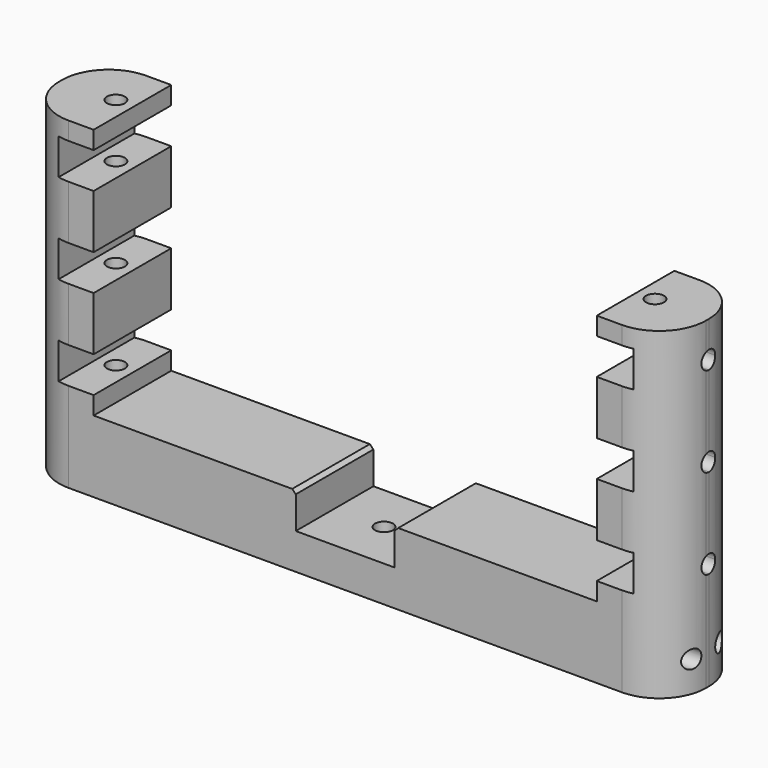
from build123d import *

# Parameters (mm, degrees)
F0_W         = 180
F0_H         = 90
F1_DEPTH     = 27
F2_W         = 140
F2_H         = 70
F3_DEPTH     = 27.001
F4_W         = 10
F4_H         = 10
F5_DEPTH     = 27.001
F6_R         = 2.5
F7_DEPTH     = 80
F9_DEPTH     = 180.001
F11_R        = 2.5
F12_DEPTH    = 20
F10_R        = 2.5
F13_DEPTH    = 20
F14_T1_DEPTH = 155
F15_W        = 27.5
F15_H        = 10
F16_DEPTH    = 27.0010001
F18_SIZE     = 1
F19_R        = 2.5
F20_DEPTH    = 90.0010001


# Not quite as in the source:
# - a fillet or chamfer that OpenCascade refuses, or shapes differently, is made with other operations: its cross-section is extruded or revolved along the edge and cut away or added


with BuildPart() as f1:
    # F0 (on Front) → F1 (new body)
    with BuildSketch(Plane.XZ):
        with Locations((90, 45)):
            Rectangle(F0_W, F0_H)
    extrude(amount=F1_DEPTH)

    # F2 (on Front) → F3 (cut, through all)
    with BuildSketch(Plane.XZ):
        with Locations((90, 55)):
            Rectangle(F2_W, F2_H)
    extrude(amount=F3_DEPTH, mode=Mode.SUBTRACT)

    # F4 (on Front) → F5 (cut, through all)
    with BuildSketch(Plane.XZ):
        with Locations((165, 80)):
            Rectangle(F4_W, F4_H)
        with Locations((165, 55)):
            Rectangle(F4_W, F4_H)
        with Locations((165, 30)):
            Rectangle(F4_W, F4_H)
        with Locations((15, 30)):
            Rectangle(F4_W, F4_H)
        with Locations((15, 55)):
            Rectangle(F4_W, F4_H)
        with Locations((15, 80)):
            Rectangle(F4_W, F4_H)
    extrude(amount=F5_DEPTH, mode=Mode.SUBTRACT)

    # F6 (on face) → F7 (cut)
    with BuildSketch(Plane.XY.offset(90)):
        with Locations((165, -13)):
            Circle(F6_R)
        with Locations((15, -13)):
            Circle(F6_R)
    extrude(amount=-F7_DEPTH, mode=Mode.SUBTRACT)

    # F8 (on Right) → F9 (cut, through all)
    with BuildSketch(Plane.YZ):
        with BuildLine():
            Line((-13, 77.5), (-13, 82.5))
            ThreePointArc((-13, 82.5), (-15.5, 80), (-13, 77.5))
        make_face()
        with BuildLine():
            ThreePointArc((-13, 77.5), (-11.232233047, 78.232233047), (-10.5, 80))
            ThreePointArc((-10.5, 80), (-11.232233047, 81.767766953), (-13, 82.5))
            Line((-13, 82.5), (-13, 77.5))
        make_face()
        with BuildLine():
            Line((-13, 52.5), (-13, 57.5))
            ThreePointArc((-13, 57.5), (-15.5, 55), (-13, 52.5))
        make_face()
        with BuildLine():
            ThreePointArc((-10.5, 55), (-11.232233047, 56.767766953), (-13, 57.5))
            Line((-13, 57.5), (-13, 52.5))
            ThreePointArc((-13, 52.5), (-11.232233047, 53.232233047), (-10.5, 55))
        make_face()
        with BuildLine():
            Line((-13, 27.5), (-13, 32.5))
            ThreePointArc((-13, 32.5), (-15.5, 30), (-13, 27.5))
        make_face()
        with BuildLine():
            ThreePointArc((-10.5, 30), (-11.232233047, 31.767766953), (-13, 32.5))
            Line((-13, 32.5), (-13, 27.5))
            ThreePointArc((-13, 27.5), (-11.232233047, 28.232233047), (-10.5, 30))
        make_face()
    extrude(amount=F9_DEPTH, mode=Mode.SUBTRACT)

    # F11 (on face) → F12 (cut)
    with BuildSketch(Plane.YZ.offset(180)):
        with Locations((-8, 8.5)):
            Circle(F11_R)
        with Locations((-18, 8.5)):
            Circle(F11_R)
    extrude(amount=-F12_DEPTH, mode=Mode.SUBTRACT)

    # F10 (on Right) → F13 (cut)
    with BuildSketch(Plane.YZ):
        with Locations((-8, 8.5)):
            Circle(F10_R)
        with Locations((-18, 8.5)):
            Circle(F10_R)
    extrude(amount=F13_DEPTH, mode=Mode.SUBTRACT)

    # F14: fillet of radius 13 on 4 edges, made by hand

    # F14_s2 → F14_t1 (cut)
    with BuildSketch(Plane.XY.offset(-32.5)):
        with BuildLine():
            ThreePointArc((0, -13), (3.8076118446, -3.8076118446), (13, 0))
            Line((13, 0), (0, 0))
            Line((0, 0), (0, -13))
        make_face()
        with BuildLine():
            ThreePointArc((0, -14), (3.8076118446, -23.1923881554), (13, -27))
            Line((13, -27), (0, -27))
            Line((0, -27), (0, -14))
        make_face()
        with BuildLine():
            ThreePointArc((167, -27), (176.1923881554, -23.1923881554), (180, -14))
            Line((180, -14), (180, -27))
            Line((180, -27), (167, -27))
        make_face()
        with BuildLine():
            ThreePointArc((167, 0), (176.1923881554, -3.8076118446), (180, -13))
            Line((180, -13), (180, 0))
            Line((180, 0), (167, 0))
        make_face()
    extrude(amount=F14_T1_DEPTH, mode=Mode.SUBTRACT)

    # F15 (on face) → F16 (cut, through all)
    with BuildSketch(Plane.XZ.offset(27)):
        with Locations((90, 15)):
            Rectangle(F15_W, F15_H)
    extrude(amount=-F16_DEPTH, mode=Mode.SUBTRACT)

    # F18
    f18_edges = [f1.edges().sort_by_distance(p)[0] for p in [
        (103.75, -13.5, 20),
        (76.25, -13.5, 20),
    ]]
    chamfer(f18_edges, length=F18_SIZE)

    # F19 (on face) → F20 (cut, through all)
    with BuildSketch(Plane(origin=(0, 0, 0), x_dir=(1, 0, 0), z_dir=(0, 0, -1))):
        with Locations((90, 13.5)):
            Circle(F19_R)
    extrude(amount=-F20_DEPTH, mode=Mode.SUBTRACT)


solid = f1.part
